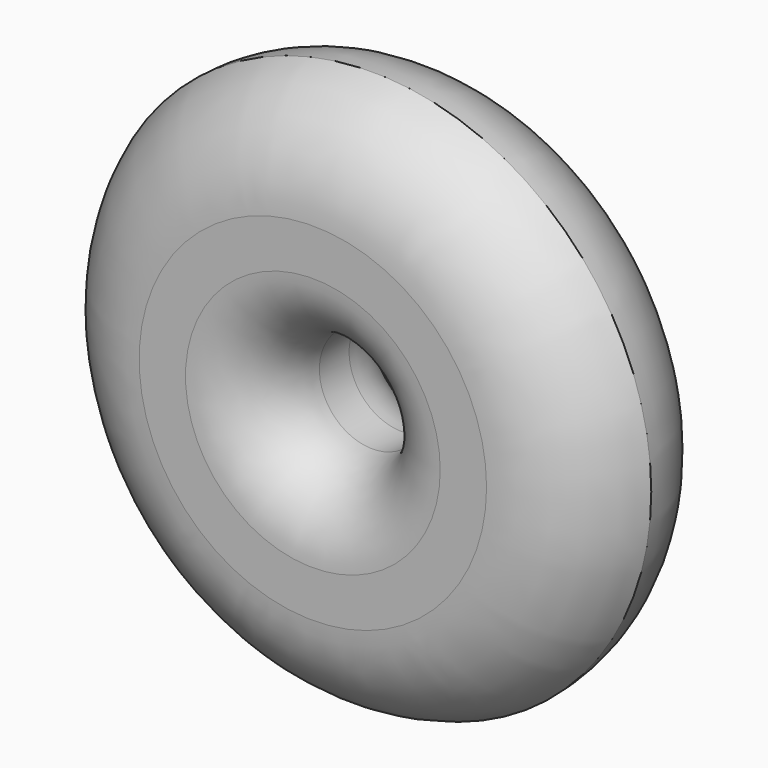
from build123d import *

# Parameters (mm, degrees)
F0_R     = 7.5
F0_R_2   = 1.425
F1_DEPTH = 5
F2_R     = 3
F4_R     = 2


# Not quite as in the source:
# - a fillet or chamfer that OpenCascade refuses, or shapes differently, is made with other operations: its cross-section is extruded or revolved along the edge and cut away or added


with BuildPart() as f1:
    # F0 (on Front) → F1 (new body)
    with BuildSketch(Plane.XZ):
        Circle(F0_R)
        Circle(F0_R_2, mode=Mode.SUBTRACT)
    extrude(amount=F1_DEPTH)

    # F2
    f2_edges = [f1.edges().sort_by_distance(p)[0] for p in [
        (-7.5, 0, 0),
    ]]
    fillet(f2_edges, radius=F2_R)

    # F3: fillet of radius 3 on 1 edges, made by hand

    # F3_s1 → F3_t2 (revolve, cut)
    with BuildSketch(Plane.XY):
        with BuildLine():
            ThreePointArc((7.5, -3), (6.4036236828, -4.4494897428), (4.6715728753, -5))
            Line((4.6715728753, -5), (7.5, -5))
            Line((7.5, -5), (7.5, -3))
        make_face()
    revolve(axis=Axis((0, -5, 0), (0, -1, 0)), mode=Mode.SUBTRACT)

    # F4
    f4_edges = [f1.edges().sort_by_distance(p)[0] for p in [
        (1.425, -2.5, 0),
        (-1.425, 0, 0),
        (-1.425, -5, 0),
    ]]
    fillet(f4_edges, radius=F4_R)


solid = f1.part
